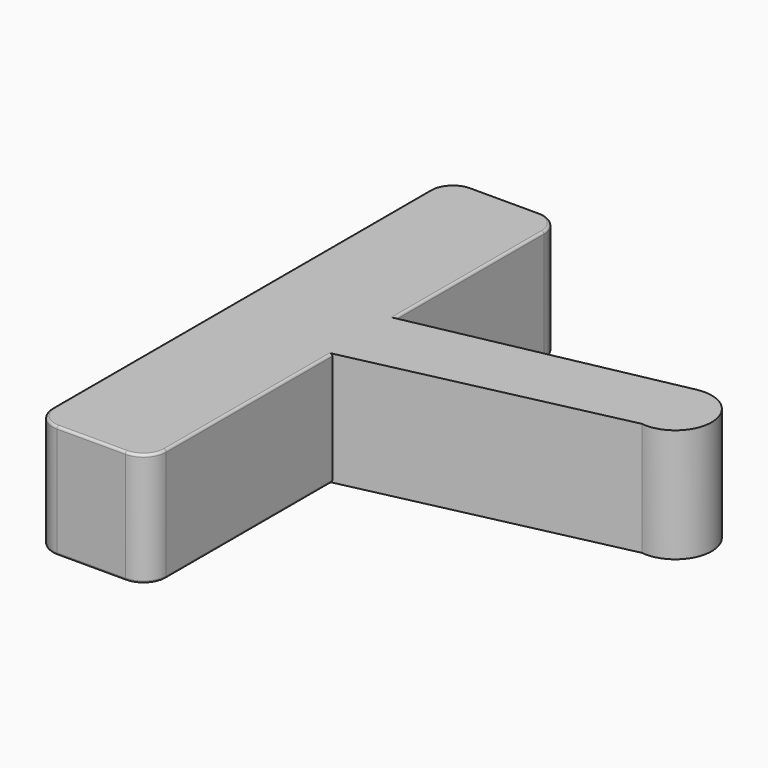
from build123d import *

# Parameters (mm, degrees)
F1_DEPTH = 25
F4_R     = 0.5311269837
F5_R     = 0.5


# Not quite as in the source:
# - the program builds the solid bodies; features that only make, move or delete a surface that nothing else refers to are left out


with BuildPart() as f1:
    # F0 (on Top) → F1 (new body)
    with BuildSketch(Plane.XY):
        with BuildLine():
            Line((27.2940341383, 7.6065342873), (-29.9786943942, -4.0269889869))
            Line((-29.9786943942, -4.0269889869), (-29.9786943942, -21.0298318416))
            Line((-29.9786943942, -21.0298318416), (27.8906263411, -8.2031255588))
            ThreePointArc((27.8906263411, -8.2031255588), (36.9003542168, 0.052951297), (27.2940341383, 7.6065342873))
        make_face()
        with BuildLine():
            Line((-34.9786943942, 42.2088094056), (-50.0355128944, 42.2088094056))
            ThreePointArc((-50.0355128944, 42.2088094056), (-53.5710468003, 40.7443433115), (-55.0355128944, 37.2088094056))
            Line((-55.0355128944, 37.2088094056), (-55.0355128944, -66.7400610447))
            ThreePointArc((-55.0355128944, -66.7400610447), (-53.5710468003, -70.2755949506), (-50.0355128944, -71.7400610447))
            Line((-50.0355128944, -71.7400610447), (-34.9786943942, -71.7400610447))
            ThreePointArc((-34.9786943942, -71.7400610447), (-31.4431604883, -70.2755949506), (-29.9786943942, -66.7400610447))
            Line((-29.9786943942, -66.7400610447), (-29.9786943942, -21.0298318416))
            Line((-29.9786943942, -21.0298318416), (-29.9786943942, -4.0269889869))
            Line((-29.9786943942, -4.0269889869), (-29.9786943942, 37.2088094056))
            ThreePointArc((-29.9786943942, 37.2088094056), (-31.4431604883, 40.7443433115), (-34.9786943942, 42.2088094056))
        make_face()
    extrude(amount=F1_DEPTH)

    # F4
    f4_edges = [f1.edges().sort_by_distance(p)[0] for p in [
        (-29.978694, -43.884946, 25),
    ]]
    fillet(f4_edges, radius=F4_R)

    # F5
    f5_edges = [f1.edges().sort_by_distance(p)[0] for p in [
        (-29.978694, -43.884946, 0),
    ]]
    fillet(f5_edges, radius=F5_R)


solid = f1.part
